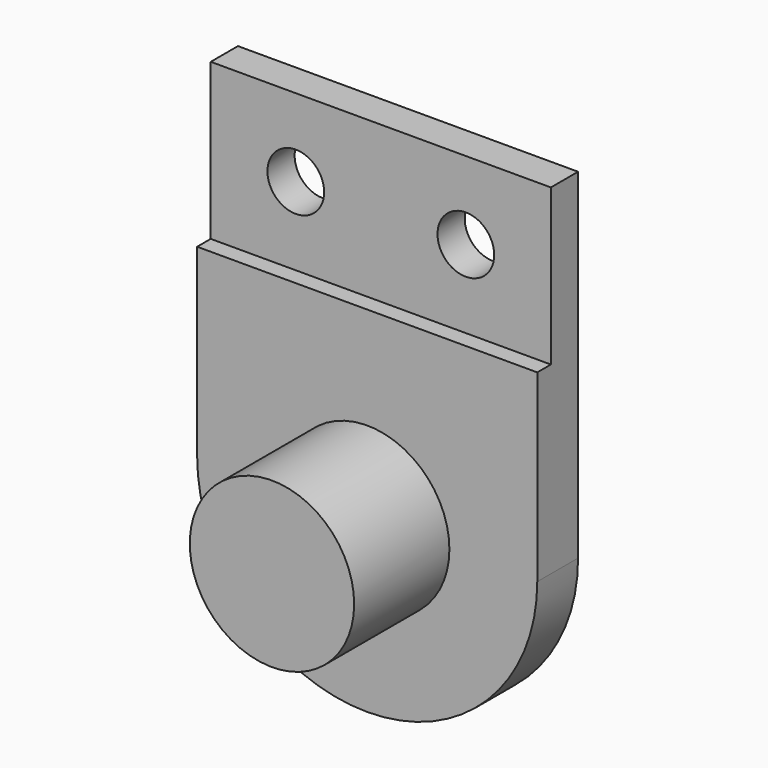
from build123d import *

# Parameters (mm, degrees)
F0_W     = 12
F0_H     = 18
F1_DEPTH = 1.8
F2_R     = 5.99999
F3_W     = 12
F3_H     = 5.5
F4_DEPTH = 0.6
F5_R     = 2.9
F6_DEPTH = 4.2
F7_R     = 1
F8_DEPTH = 25


# Not quite as in the source:
# - a fillet or chamfer is up to 0.001 mm smaller than in the source, because OpenCascade refuses the exact size


with BuildPart() as f1:
    # F0 (on Front) → F1 (new body)
    with BuildSketch(Plane.XZ):
        Rectangle(F0_W, F0_H)
    extrude(amount=F1_DEPTH)

    # F2 (radius 6 in the source; OpenCascade refuses exactly that, so slightly less here)
    f2_edges = [f1.edges().sort_by_distance(p)[0] for p in [
        (6, -0.9, -9),
        (-6, -0.9, -9),
    ]]
    fillet(f2_edges, radius=F2_R)

    # F3 (on face) → F4 (cut)
    with BuildSketch(Plane.XZ.offset(1.8)):
        with Locations((0, 6.25)):
            Rectangle(F3_W, F3_H)
    extrude(amount=-F4_DEPTH, mode=Mode.SUBTRACT)

    # F5 (on face) → F6 (join)
    with BuildSketch(Plane.XZ.offset(1.8)):
        with Locations((0, -3)):
            Circle(F5_R)
    extrude(amount=F6_DEPTH)

    # F7 (on face) → F8 (cut)
    with BuildSketch(Plane.XZ.offset(1.2)):
        with Locations((-3, 6.25)):
            Circle(F7_R)
        with Locations((3, 6.25)):
            Circle(F7_R)
    extrude(amount=-F8_DEPTH, mode=Mode.SUBTRACT)


solid = f1.part
